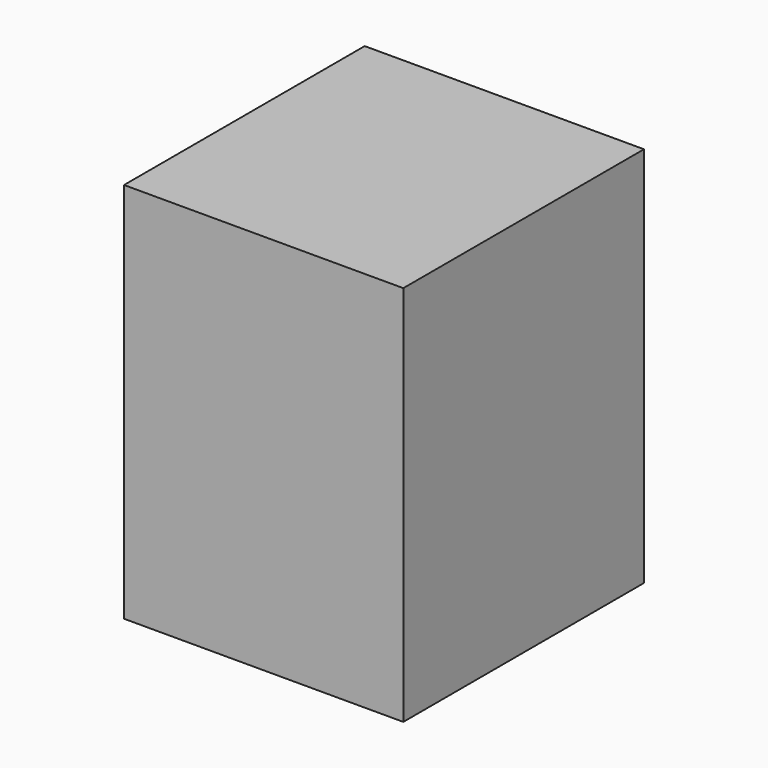
from build123d import *

# Parameters (mm, degrees)
F1_W     = 11.7906006053
F1_H     = 16.1216966808
F3_DEPTH = 12.7


# Not quite as in the source:
# - the program builds the solid bodies; features that only make, move or delete a surface that nothing else refers to are left out


with BuildPart() as f3:
    # F1 (on Front) → F3 (new body)
    with BuildSketch(Plane.XZ):
        with Locations((-16.8220824562, 20.3086268157)):
            Rectangle(F1_W, F1_H)
    extrude(amount=F3_DEPTH)


solid = f3.part
